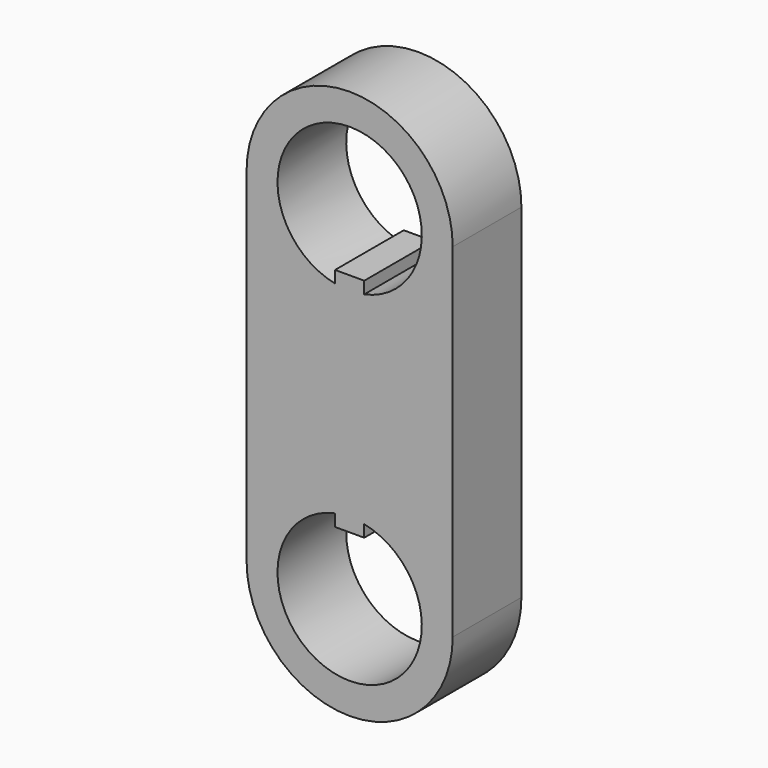
from build123d import *

# Parameters (mm, degrees)
F0_R     = 4.2
F1_DEPTH = 5
F3_DEPTH = 5


# Not quite as in the source:
# - a pattern or mirror of a feature is missing from the dataset's text; its kind, count and spacing are read off the source's solid


with BuildPart() as f1:
    # F0 (on Front) → F1 (new body)
    with BuildSketch(Plane.XZ):
        with BuildLine():
            Line((-6, 20), (-6, 0))
            ThreePointArc((-6, 0), (0, -6), (6, 0))
            Line((6, 0), (6, 20))
            ThreePointArc((6, 20), (0, 26), (-6, 20))
        make_face()
        Circle(F0_R, mode=Mode.SUBTRACT)
        with Locations((0, 20)):
            Circle(F0_R, mode=Mode.SUBTRACT)
    extrude(amount=F1_DEPTH)

    # F2 (on face) → F3 (join, through all)
    with BuildSketch(Plane.XZ.offset(5)):
        Polygon((-0.85, 16.5869111364), (-0.85, 15.8869111364), (0, 14.8420017213), (0.85, 15.8869111364), (0.85, 16.5869111364), align=None)
    f3 = extrude(amount=-F3_DEPTH)

    # F3_copies: F3 across plane
    add(f3.mirror(Plane(origin=(0, 0, 10), x_dir=(-1, 0, 0), z_dir=(0, 0, -1))))


solid = f1.part
